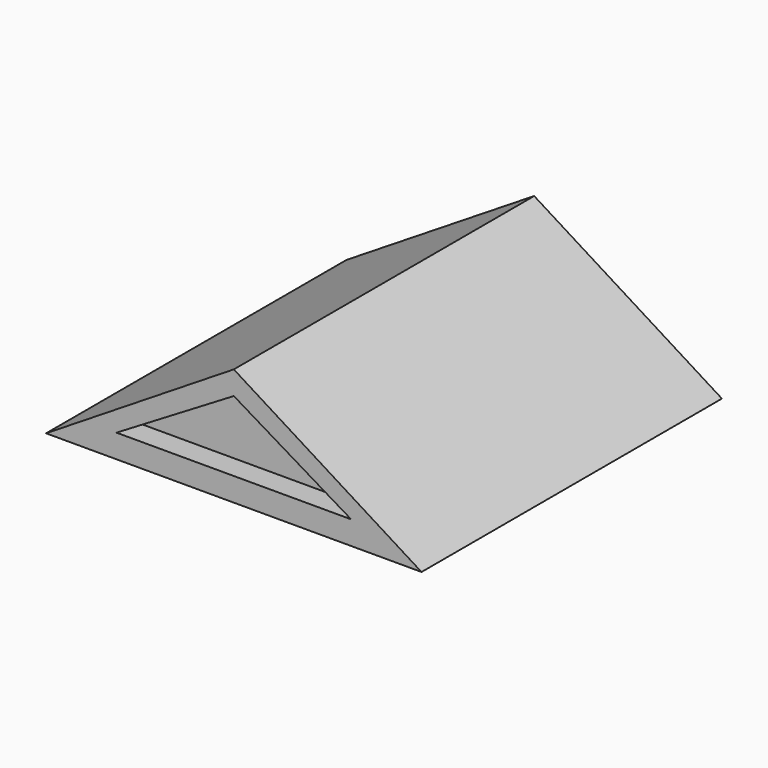
from build123d import *

# Parameters (mm, degrees)
F1_DEPTH = 177.8
F2_DEPTH = 177.8
F3_DEPTH = 203.2
F4_DEPTH = 203.2


with BuildPart() as f1:
    # F0 (on Front) → F1 (new body)
    with BuildSketch(Plane.XZ):
        Polygon((-127, 0), (0, 0), (0, 76.2), align=None)
        Polygon((0, 76.2), (0, 0), (127, 0), align=None)
    extrude(amount=F1_DEPTH)

    # F2 (add): a face of the model
    f2_faces = [f1.faces().sort_by_distance(p)[0] for p in [
        (0, 0, 25.4),
    ]]
    extrude(f2_faces, amount=F2_DEPTH)

    # F0 (on Front) → F3 (join)
    with BuildSketch(Plane.XZ):
        Polygon((0, 101.6), (-203.2, -25.4), (203.2, -25.4), align=None)
        Polygon((127, 0), (0, 0), (-127, 0), (0, 76.2), align=None, mode=Mode.SUBTRACT)
    extrude(amount=F3_DEPTH)

    # F0 (on Front) → F4 (join)
    with BuildSketch(Plane.XZ):
        Polygon((0, 101.6), (-203.2, -25.4), (203.2, -25.4), align=None)
        Polygon((127, 0), (0, 0), (-127, 0), (0, 76.2), align=None, mode=Mode.SUBTRACT)
    extrude(amount=-F4_DEPTH)


solid = f1.part
